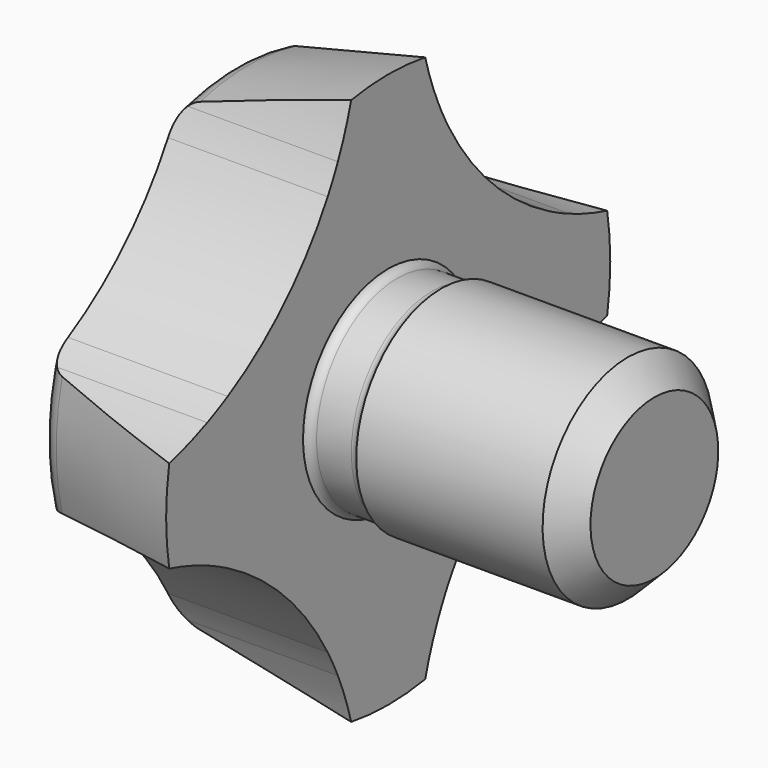
from build123d import *

# Parameters (mm, degrees)
F0_W     = 3.5
F0_H     = 2
F0_W_2   = 0.65359
F0_H_2   = 1.9
F3_DEPTH = 25


# Not quite as in the source:
# - ends of sketch curves that miss each other by under 0.0002 mm in the source are joined


with BuildPart() as f1:
    # F0 (on Front) → F1 (revolve)
    with BuildSketch(Plane.XZ):
        with BuildLine():
            ThreePointArc((6.2807068037, 4.5095537326), (6.0134401175, 4.3309714378), (5.910117, 4.026591))
            Line((5.910117, 4.026591), (5.910117, 0))
            Line((5.910117, 0), (8.910117, 0))
            Line((8.910117, 0), (8.910117, 1.999999965))
            Line((8.910117, 1.999999965), (8.910117, 5.214102))
            Line((8.910117, 5.214102), (6.2807068037, 4.5095537326))
        make_face()
        with BuildLine():
            Line((9.736912, 1.9), (9.736912, 0))
            Line((9.736912, 0), (9.910117, 0))
            Line((9.910117, 0), (9.910117, 2))
            ThreePointArc((9.9101170606, 1.999999965), (9.8369119825, 1.9267949091), (9.736912, 1.9))
        make_face()
        with Locations((11.660117, 1)):
            Rectangle(F0_W, F0_H)
        with Locations((9.410117, 0.95)):
            Rectangle(F0_W_2, F0_H_2)
        with BuildLine():
            Line((8.910117, 1.999999965), (8.910117, 0))
            Line((8.910117, 0), (9.083322, 0))
            Line((9.083322, 0), (9.083322, 1.9))
            ThreePointArc((9.083322, 1.9), (8.9833220175, 1.9267949091), (8.9101169394, 1.999999965))
        make_face()
        Polygon((13.410117, 2), (13.410117, 0), (13.910117, 0), (13.910117, 1.5), align=None)
    revolve(axis=Axis((10.414001145, 0, 0), (-1, 0, 0)))

    # F2 (on face) → F3 (cut)
    with BuildSketch(Plane(origin=(5.910117, 0, 0), x_dir=(0, -1, 0), z_dir=(-1, 0, 0))):
        with BuildLine():
            ThreePointArc((1.1816228772, -4.2490125583), (1.0079083628, -4.6889045584), (0.8693810599, -5.1411123543))
            ThreePointArc((0.8693810599, -5.1411123543), (3.686926882, -3.686926882), (5.1411123543, -0.8693810599))
            ThreePointArc((5.1411123543, -0.8693810599), (4.6889045584, -1.0079083628), (4.2490125583, -1.1816228772))
            ThreePointArc((4.2490125583, -1.1816228772), (4.0057430921, -1.2955299839), (3.7678156951, -1.420211241))
            ThreePointArc((3.7678156951, -1.420211241), (2.8472298012, -2.8472298012), (1.420211241, -3.7678156951))
            ThreePointArc((1.420211241, -3.7678156951), (1.2955299839, -4.0057430921), (1.1816228772, -4.2490125583))
        make_face()
        with BuildLine():
            ThreePointArc((-5.1411123543, -0.8693810599), (-3.686926882, -3.686926882), (-0.8693810599, -5.1411123543))
            ThreePointArc((-0.8693810599, -5.1411123543), (-1.0079083664, -4.6889048876), (-1.1816228201, -4.2490132008))
            ThreePointArc((-1.1816228201, -4.2490132008), (-1.2955301515, -4.0057433246), (-1.4202116652, -3.7678155352))
            ThreePointArc((-1.4202116652, -3.7678155352), (-2.8472298012, -2.8472298012), (-3.7678155352, -1.4202116652))
            ThreePointArc((-3.7678155352, -1.4202116652), (-4.0057429748, -1.2955303249), (-4.2490124865, -1.1816231353))
            ThreePointArc((-4.2490124865, -1.1816231353), (-4.6889045191, -1.0079084953), (-5.1411123543, -0.8693810599))
        make_face()
        with BuildLine():
            ThreePointArc((4.2490125583, 1.1816228772), (4.6889045584, 1.0079083628), (5.1411123543, 0.8693810599))
            ThreePointArc((5.1411123543, 0.8693810599), (3.686926882, 3.686926882), (0.8693810599, 5.1411123543))
            ThreePointArc((0.8693810599, 5.1411123543), (1.0079083628, 4.6889045584), (1.1816228772, 4.2490125583))
            ThreePointArc((1.1816228772, 4.2490125583), (1.2955299839, 4.0057430921), (1.420211241, 3.7678156951))
            ThreePointArc((1.420211241, 3.7678156951), (2.8472298012, 2.8472298012), (3.7678156951, 1.420211241))
            ThreePointArc((3.7678156951, 1.420211241), (4.0057430921, 1.2955299839), (4.2490125583, 1.1816228772))
        make_face()
        with BuildLine():
            ThreePointArc((3.7678156951, -1.420211241), (2.4284046412, -2.4284046412), (1.420211241, -3.7678156951))
            ThreePointArc((1.420211241, -3.7678156951), (2.8472298012, -2.8472298012), (3.7678156951, -1.420211241))
        make_face()
        with BuildLine():
            ThreePointArc((-0.8693810599, 5.1411123543), (-3.686926882, 3.686926882), (-5.1411123543, 0.8693810599))
            ThreePointArc((-5.1411123543, 0.8693810599), (-4.6889043312, 1.0079080153), (-4.2490121021, 1.1816222641))
            ThreePointArc((-4.2490121021, 1.1816222641), (-4.0057431642, 1.295528931), (-3.7678162701, 1.4202097156))
            ThreePointArc((-3.7678162701, 1.4202097156), (-2.8472298012, 2.8472298012), (-1.4202097156, 3.7678162701))
            ThreePointArc((-1.4202097156, 3.7678162701), (-1.2955287576, 4.0057435139), (-1.181621949, 4.2490128164))
            ThreePointArc((-1.181621949, 4.2490128164), (-1.0079078864, 4.6889046997), (-0.8693810599, 5.1411123543))
        make_face()
        with BuildLine():
            ThreePointArc((-3.7678155352, -1.4202116652), (-2.8472298012, -2.8472298012), (-1.4202116652, -3.7678155352))
            ThreePointArc((-1.4202116652, -3.7678155352), (-2.4284049327, -2.4284049327), (-3.7678155352, -1.4202116652))
        make_face()
        with BuildLine():
            ThreePointArc((1.420211241, 3.7678156951), (2.4284046412, 2.4284046412), (3.7678156951, 1.420211241))
            ThreePointArc((3.7678156951, 1.420211241), (2.8472298012, 2.8472298012), (1.420211241, 3.7678156951))
        make_face()
        with BuildLine():
            ThreePointArc((-1.4202097156, 3.7678162701), (-2.8472298012, 2.8472298012), (-3.7678162701, 1.4202097156))
            ThreePointArc((-3.7678162701, 1.4202097156), (-2.428403593, 2.428403593), (-1.4202097156, 3.7678162701))
        make_face()
    extrude(amount=-F3_DEPTH, mode=Mode.SUBTRACT)


solid = f1.part
